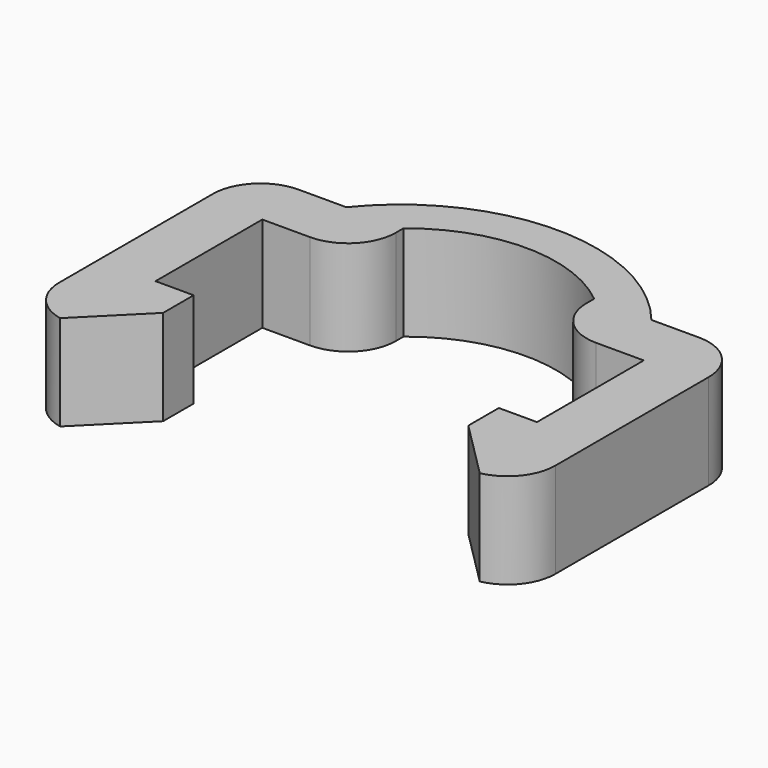
from build123d import *

# Parameters (mm, degrees)
F1_DEPTH    = 5
F2_SIZE     = 3
F3_T1_DEPTH = 17.2474487139
F3_T3_DEPTH = 17.5


# Not quite as in the source:
# - a fillet or chamfer that OpenCascade refuses, or shapes differently, is made with other operations: its cross-section is extruded or revolved along the edge and cut away or added
# - a feature names something its author has since deleted; it is built from what else it names


with BuildPart() as f1:
    # F0 (on Top) → F1 (new body)
    with BuildSketch(Plane.XY):
        with BuildLine():
            Line((-13, 12), (-13, 0))
            Line((-13, 0), (-10, 0))
            Line((-10, 0), (-8, 0))
            Line((-8, 0), (-8, 5))
            Line((-8, 5), (-10, 5))
            Line((-10, 5), (-10, 12))
            Line((-10, 12), (-5, 12))
            Line((-5, 12), (-5, 15))
            ThreePointArc((-5, 15), (0, 16.7884008853), (5, 15))
            Line((5, 15), (5, 12))
            Line((5, 12), (10, 12))
            Line((10, 12), (10, 5))
            Line((10, 5), (8, 5))
            Line((8, 5), (8, 0))
            Line((8, 0), (10, 0))
            Line((10, 0), (13, 0))
            Line((13, 0), (13, 15))
            Line((13, 15), (10, 15))
            Line((10, 15), (8, 15))
            ThreePointArc((8, 15), (0, 18.8196946698), (-8, 15))
            Line((-8, 15), (-10, 15))
            Line((-10, 15), (-13, 15))
            Line((-13, 15), (-13, 12))
        make_face()
    extrude(amount=F1_DEPTH)

    # F2
    f2_edges = [f1.edges().sort_by_distance(p)[0] for p in [
        (-8, 0, 2.5),
        (8, 0, 2.5),
    ]]
    chamfer(f2_edges, length=F2_SIZE)

    # F3: fillet of radius 2.5 on 6 edges, made by hand

    # F3_s2 → F3_t1 (cut)
    with BuildSketch(Plane.XY.offset(-6.123724357)):
        with BuildLine():
            ThreePointArc((-11, 0), (-12.4364916731, 0.8683509127), (-13, 2.4494897428))
            Line((-13, 2.4494897428), (-13, 0))
            Line((-13, 0), (-11, 0))
        make_face()
        with BuildLine():
            ThreePointArc((13, 2.4494897428), (12.4364916731, 0.8683509127), (11, 0))
            Line((11, 0), (13, 0))
            Line((13, 0), (13, 2.4494897428))
        make_face()
    extrude(amount=F3_T1_DEPTH, mode=Mode.SUBTRACT)

    # F3_s4 → F3_t3 (cut)
    with BuildSketch(Plane.XY.offset(-6.25)):
        with BuildLine():
            ThreePointArc((-13, 12.5), (-12.267766953, 14.267766953), (-10.5, 15))
            Line((-10.5, 15), (-13, 15))
            Line((-13, 15), (-13, 12.5))
        make_face()
        with BuildLine():
            ThreePointArc((10.5, 15), (12.267766953, 14.267766953), (13, 12.5))
            Line((13, 12.5), (13, 15))
            Line((13, 15), (10.5, 15))
        make_face()
        with BuildLine():
            ThreePointArc((-7.5, 12), (-5.732233047, 12.732233047), (-5, 14.5))
            Line((-5, 14.5), (-5, 12))
            Line((-5, 12), (-7.5, 12))
        make_face()
        with BuildLine():
            ThreePointArc((5, 14.5), (5.732233047, 12.732233047), (7.5, 12))
            Line((7.5, 12), (5, 12))
            Line((5, 12), (5, 14.5))
        make_face()
    extrude(amount=F3_T3_DEPTH, mode=Mode.SUBTRACT)


solid = f1.part
